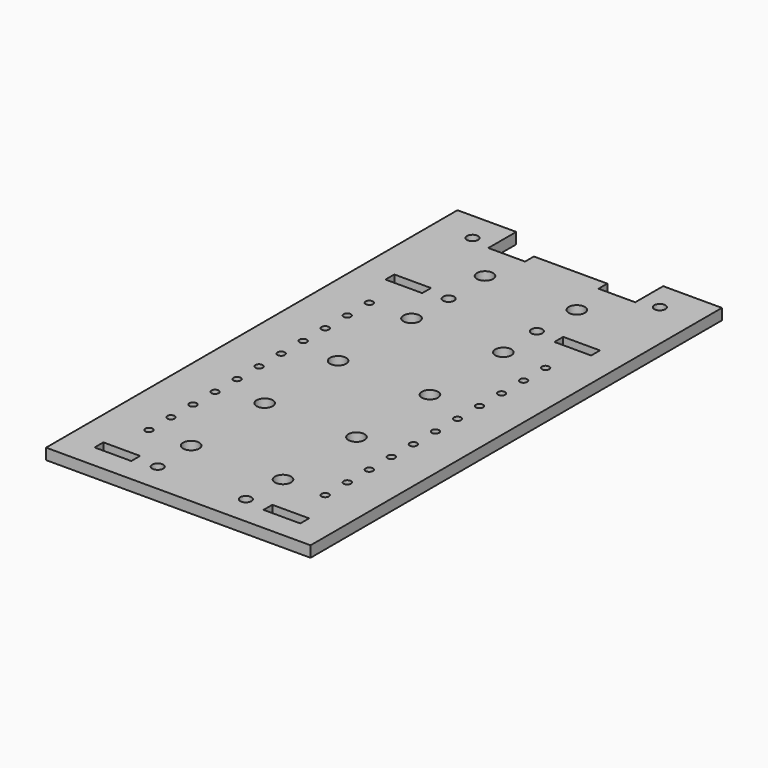
from build123d import *

# Parameters (mm, degrees)
F1_W     = 10
F1_H     = 3
F2_DEPTH = 3
F4_D     = 2
F6_D     = 3
F8_D     = 4.4


# Not quite as in the source:
# - a feature names something its author has since deleted; it is built from what else it names


with BuildPart() as f2:
    # F1 (on Top) → F2 (new body)
    with BuildSketch(Plane.XY):
        Polygon((-36, -70), (36, -70), (36, 70), (20, 70), (20, 63.5), (20, 60.5), (10, 60.5), (10, 63.5), (-10, 63.5), (-10, 60.5), (-20, 60.5), (-20, 63.5), (-20, 70), (-36, 70), align=None)
        with Locations((-23, -62)):
            Rectangle(F1_W, F1_H, mode=Mode.SUBTRACT)
        with Locations((23, -62)):
            Rectangle(F1_W, F1_H, mode=Mode.SUBTRACT)
        with Locations((-23, 37)):
            Rectangle(F1_W, F1_H, mode=Mode.SUBTRACT)
        with Locations((23, 37)):
            Rectangle(F1_W, F1_H, mode=Mode.SUBTRACT)
    extrude(amount=F2_DEPTH)

    # F4 (through all)
    with Locations(Plane.XY.offset(3)):
        with Locations((24, -50), (24, -42.5), (24, -35), (-24, -50), (-24, -42.5), (-24, -35), (-24, -27.5), (24, -27.5), (-24, -20), (24, -20), (-24, -12.5), (-24, -5), (-24, 2.5), (-24, 10), (-24, 17.5), (24, -12.5), (24, -5), (24, 2.5), (24, 10), (24, 17.5), (-24, 25), (24, 25)):
            Hole(F4_D / 2)

    # F6 (through all)
    with Locations(Plane(origin=(0, 0, 0), x_dir=(1, 0, 0), z_dir=(0, 0, -1))):
        with Locations((-25.5, -62), (25.5, -62), (-12, 62), (12, 62), (-12, -37), (12, -37)):
            Hole(F6_D / 2)

    # F8 (through all)
    with Locations(Plane.XY.offset(3)):
        with Locations((-12.5, -50), (12.5, -50), (-12.5, -25), (12.5, -25), (-12.5, 0), (12.5, 0), (-12.5, 25), (12.5, 25), (-12.5, 50), (12.5, 50)):
            Hole(F8_D / 2)


solid = f2.part
